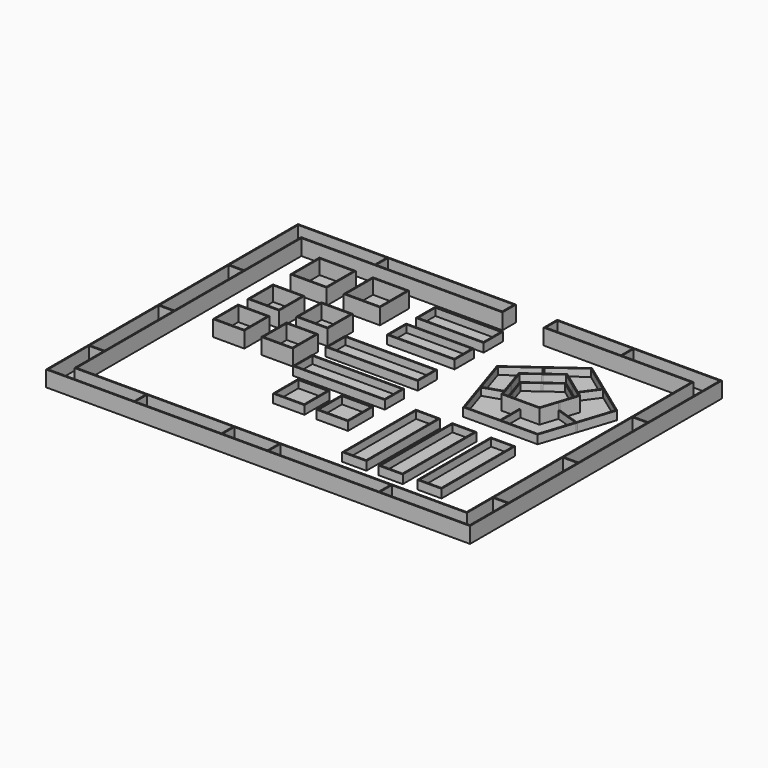
from build123d import *

# Parameters (mm, degrees)
F1_W     = 14
F1_H     = 14
F3_DEPTH = 6
F1_W_2   = 12
F1_H_2   = 12
F0_W     = 6
F0_H     = 0.5
F0_W_2   = 0.5
F0_H_2   = 6
F0_H_3   = 35.5
F0_W_3   = 52
F0_W_4   = 35.5
F0_W_5   = 18.5
F0_W_6   = 45.5
F0_W_7   = 31
F4_T     = 0.5
F4_2_T   = 0.5
F4_3_T   = 0.5
F4_4_T   = 0.5
F4_5_T   = 0.5
F4_6_T   = 0.5
F4_7_T   = 0.5
F4_8_T   = 0.5
F1_W_3   = 27
F1_H_3   = 9
F5_DEPTH = 3
F1_W_4   = 37
F1_W_5   = 9
F1_H_4   = 37
F2_W     = 0.5
F2_H     = 10.322864
F6_T     = 0.5
F6_2_T   = 0.5
F6_3_T   = 0.5
F6_4_T   = 0.5
F6_5_T   = 0.5
F6_6_T   = 0.5
F6_7_T   = 0.5
F6_8_T   = 0.5
F6_9_T   = 0.5
F6_10_T  = 0.5
F7_DEPTH = 6
F8_DEPTH = 3


with BuildPart() as f3:
    # F1 (on Top) → F3 (new body)
    with BuildSketch(Plane.XY):
        with Locations((-36.439199, 38.914477)):
            Rectangle(F1_W, F1_H)
    extrude(amount=F3_DEPTH)

    # F4#3
    f4_3_openings = [f3.faces().sort_by_distance(p)[0] for p in [
        (-36.439199, 38.914477, 6),
    ]]
    offset(amount=F4_3_T, openings=f4_3_openings, kind=Kind.INTERSECTION)


with BuildPart() as f3b:
    # F1 (on Top) → F3, piece 2 (new body)
    with BuildSketch(Plane.XY):
        with Locations((-58.439199, 38.914477)):
            Rectangle(F1_W, F1_H)
    extrude(amount=F3_DEPTH)

    # F4#2
    f4_2_openings = [f3b.faces().sort_by_distance(p)[0] for p in [
        (-58.439199, 38.914477, 6),
    ]]
    offset(amount=F4_2_T, openings=f4_2_openings, kind=Kind.INTERSECTION)


with BuildPart() as f3c:
    # F1 (on Top) → F3, piece 3 (new body)
    with BuildSketch(Plane.XY):
        with Locations((-59.439199, 15.914477)):
            Rectangle(F1_W_2, F1_H_2)
    extrude(amount=F3_DEPTH)

    # F4#5
    f4_5_openings = [f3c.faces().sort_by_distance(p)[0] for p in [
        (-59.439199, 15.914477, 6),
    ]]
    offset(amount=F4_5_T, openings=f4_5_openings, kind=Kind.INTERSECTION)


with BuildPart() as f3d:
    # F1 (on Top) → F3, piece 4 (new body)
    with BuildSketch(Plane.XY):
        with Locations((-59.439199, -2.085523)):
            Rectangle(F1_W_2, F1_H_2)
    extrude(amount=F3_DEPTH)

    # F4#6
    f4_6_openings = [f3d.faces().sort_by_distance(p)[0] for p in [
        (-59.439199, -2.085523, 6),
    ]]
    offset(amount=F4_6_T, openings=f4_6_openings, kind=Kind.INTERSECTION)


with BuildPart() as f3e:
    # F1 (on Top) → F3, piece 5 (new body)
    with BuildSketch(Plane.XY):
        with Locations((-39.439199, -2.085523)):
            Rectangle(F1_W_2, F1_H_2)
    extrude(amount=F3_DEPTH)

    # F4#7
    f4_7_openings = [f3e.faces().sort_by_distance(p)[0] for p in [
        (-39.439199, -2.085523, 6),
    ]]
    offset(amount=F4_7_T, openings=f4_7_openings, kind=Kind.INTERSECTION)


with BuildPart() as f3f:
    # F1 (on Top) → F3, piece 6 (new body)
    with BuildSketch(Plane.XY):
        with Locations((-39.439199, 15.914477)):
            Rectangle(F1_W_2, F1_H_2)
    extrude(amount=F3_DEPTH)

    # F4#4
    f4_4_openings = [f3f.faces().sort_by_distance(p)[0] for p in [
        (-39.439199, 15.914477, 6),
    ]]
    offset(amount=F4_4_T, openings=f4_4_openings, kind=Kind.INTERSECTION)


with BuildPart() as f3g:
    # F0 (on Top) → F3, piece 7 (new body)
    with BuildSketch(Plane.XY):
        Polygon((-48.945705, 59.870679), (-85.445705, 59.870679), (-85.445705, 24.370679), (-79.445705, 24.370679), (-79.445705, 53.870679), (-48.945705, 53.870679), align=None)
        with Locations((-82.445705, 24.120679)):
            Rectangle(F0_W, F0_H)
        with Locations((-48.695705, 56.870679)):
            Rectangle(F0_W_2, F0_H_2)
        with Locations((-82.445705, 6.120679)):
            Rectangle(F0_W, F0_H_3)
        with Locations((-22.445705, 56.870679)):
            Rectangle(F0_W_3, F0_H_2)
        with Locations((-82.445705, -11.879321)):
            Rectangle(F0_W, F0_H)
        with Locations((-82.445705, -29.879321)):
            Rectangle(F0_W, F0_H_3)
        with Locations((-82.445705, -47.879321)):
            Rectangle(F0_W, F0_H)
        Polygon((-79.445705, -48.129321), (-85.445705, -48.129321), (-85.445705, -69.129321), (-49.945705, -69.129321), (-49.945705, -63.129321), (-79.13054, -63.129321), (-79.445705, -63.129321), align=None)
        with Locations((-49.695705, -66.129321)):
            Rectangle(F0_W_2, F0_H_2)
        with Locations((-31.695705, -66.129321)):
            Rectangle(F0_W_4, F0_H_2)
        with Locations((-13.695705, -66.129321)):
            Rectangle(F0_W_2, F0_H_2)
        with Locations((-4.195705, -66.129321)):
            Rectangle(F0_W_5, F0_H_2)
        with Locations((5.304295, -66.129321)):
            Rectangle(F0_W_2, F0_H_2)
        with Locations((28.304295, -66.129321)):
            Rectangle(F0_W_6, F0_H_2)
        with Locations((51.304295, -66.129321)):
            Rectangle(F0_W_2, F0_H_2)
        Polygon((51.554295, -63.129321), (51.554295, -69.129321), (88.554295, -69.129321), (88.554295, -49.629321), (82.554295, -49.629321), (82.554295, -63.129321), align=None)
        with Locations((85.554295, -49.379321)):
            Rectangle(F0_W, F0_H)
        with Locations((85.554295, -31.379321)):
            Rectangle(F0_W, F0_H_3)
        with Locations((85.554295, -13.379321)):
            Rectangle(F0_W, F0_H)
        with Locations((85.554295, 4.620679)):
            Rectangle(F0_W, F0_H_3)
        with Locations((85.554295, 22.620679)):
            Rectangle(F0_W, F0_H)
        Polygon((82.554295, 22.870679), (88.554295, 22.870679), (88.554295, 59.870679), (53.054295, 59.870679), (53.054295, 53.870679), (82.554295, 53.870679), align=None)
        with Locations((52.804295, 56.870679)):
            Rectangle(F0_W_2, F0_H_2)
        with Locations((37.054295, 56.870679)):
            Rectangle(F0_W_7, F0_H_2)
    extrude(amount=F3_DEPTH)

    # F4
    f4_openings = [f3g.faces().sort_by_distance(p)[0] for p in [
        (-83.279671, -4.629321, 6),
    ]]
    offset(amount=F4_T, openings=f4_openings, kind=Kind.INTERSECTION)

    # F0 (on Top) → F7 (join)
    with BuildSketch(Plane.XY):
        with Locations((-48.695705, 56.870679)):
            Rectangle(F0_W_2, F0_H_2)
        with Locations((-82.445705, 24.120679)):
            Rectangle(F0_W, F0_H)
        with Locations((-82.445705, -11.879321)):
            Rectangle(F0_W, F0_H)
        with Locations((-82.445705, -47.879321)):
            Rectangle(F0_W, F0_H)
        with Locations((-49.695705, -66.129321)):
            Rectangle(F0_W_2, F0_H_2)
        with Locations((-13.695705, -66.129321)):
            Rectangle(F0_W_2, F0_H_2)
        with Locations((5.304295, -66.129321)):
            Rectangle(F0_W_2, F0_H_2)
        with Locations((51.304295, -66.129321)):
            Rectangle(F0_W_2, F0_H_2)
        with Locations((85.554295, -49.379321)):
            Rectangle(F0_W, F0_H)
        with Locations((85.554295, -13.379321)):
            Rectangle(F0_W, F0_H)
        with Locations((85.554295, 22.620679)):
            Rectangle(F0_W, F0_H)
        with Locations((52.804295, 56.870679)):
            Rectangle(F0_W_2, F0_H_2)
    extrude(amount=F7_DEPTH)


with BuildPart() as f3h:
    # F2 (on Top) → F3, piece 8 (new body)
    with BuildSketch(Plane.XY):
        Polygon((46.768948, 9.115655), (47.268948, 9.115655), (54.768948, 9.115655), (56.932067, 15.773051), (57.086575, 16.248579), (59.404203, 23.381503), (53.336575, 27.789892), (52.932067, 28.083785), (47.268948, 32.198282), (41.20132, 27.789892), (40.796812, 27.496), (35.133693, 23.381503), (37.45132, 16.248579), (37.605829, 15.773051), (39.768948, 9.115655), align=None)
    extrude(amount=F3_DEPTH)

    # F4#8
    f4_8_openings = [f3h.faces().sort_by_distance(p)[0] for p in [
        (47.268948, 19.43852, 6),
    ]]
    offset(amount=F4_8_T, openings=f4_8_openings, kind=Kind.INTERSECTION)


with BuildPart() as f5:
    # F1 (on Top) → F5 (new body)
    with BuildSketch(Plane.XY):
        with Locations((-4.939199, 42.414477)):
            Rectangle(F1_W_3, F1_H_3)
    extrude(amount=F5_DEPTH)

    # F6
    f6_openings = [f5.faces().sort_by_distance(p)[0] for p in [
        (-4.939199, 42.414477, 3),
    ]]
    offset(amount=F6_T, openings=f6_openings, kind=Kind.INTERSECTION)


with BuildPart() as f5b:
    # F1 (on Top) → F5, piece 2 (new body)
    with BuildSketch(Plane.XY):
        with Locations((-4.939199, 27.414477)):
            Rectangle(F1_W_3, F1_H_3)
    extrude(amount=F5_DEPTH)

    # F6#2
    f6_2_openings = [f5b.faces().sort_by_distance(p)[0] for p in [
        (-4.939199, 27.414477, 3),
    ]]
    offset(amount=F6_2_T, openings=f6_2_openings, kind=Kind.INTERSECTION)


with BuildPart() as f5c:
    # F1 (on Top) → F5, piece 3 (new body)
    with BuildSketch(Plane.XY):
        with Locations((-9.939199, 8.414477)):
            Rectangle(F1_W_4, F1_H_3)
    extrude(amount=F5_DEPTH)

    # F6#3
    f6_3_openings = [f5c.faces().sort_by_distance(p)[0] for p in [
        (-9.939199, 8.414477, 3),
    ]]
    offset(amount=F6_3_T, openings=f6_3_openings, kind=Kind.INTERSECTION)


with BuildPart() as f5d:
    # F1 (on Top) → F5, piece 4 (new body)
    with BuildSketch(Plane.XY):
        with Locations((-9.939199, -8.585523)):
            Rectangle(F1_W_4, F1_H_3)
    extrude(amount=F5_DEPTH)

    # F6#4
    f6_4_openings = [f5d.faces().sort_by_distance(p)[0] for p in [
        (-9.939199, -8.585523, 3),
    ]]
    offset(amount=F6_4_T, openings=f6_4_openings, kind=Kind.INTERSECTION)


with BuildPart() as f5e:
    # F1 (on Top) → F5, piece 5 (new body)
    with BuildSketch(Plane.XY):
        with Locations((-15.439199, -26.085523)):
            Rectangle(F1_W_2, F1_H_2)
    extrude(amount=F5_DEPTH)

    # F6#5
    f6_5_openings = [f5e.faces().sort_by_distance(p)[0] for p in [
        (-15.439199, -26.085523, 3),
    ]]
    offset(amount=F6_5_T, openings=f6_5_openings, kind=Kind.INTERSECTION)


with BuildPart() as f5f:
    # F1 (on Top) → F5, piece 6 (new body)
    with BuildSketch(Plane.XY):
        with Locations((2.560801, -26.085523)):
            Rectangle(F1_W_2, F1_H_2)
    extrude(amount=F5_DEPTH)

    # F6#6
    f6_6_openings = [f5f.faces().sort_by_distance(p)[0] for p in [
        (2.560801, -26.085523, 3),
    ]]
    offset(amount=F6_6_T, openings=f6_6_openings, kind=Kind.INTERSECTION)


with BuildPart() as f5g:
    # F1 (on Top) → F5, piece 7 (new body)
    with BuildSketch(Plane.XY):
        with Locations((26.060801, -31.585523)):
            Rectangle(F1_W_5, F1_H_4)
    extrude(amount=F5_DEPTH)

    # F6#7
    f6_7_openings = [f5g.faces().sort_by_distance(p)[0] for p in [
        (26.060801, -31.585523, 3),
    ]]
    offset(amount=F6_7_T, openings=f6_7_openings, kind=Kind.INTERSECTION)


with BuildPart() as f5h:
    # F1 (on Top) → F5, piece 8 (new body)
    with BuildSketch(Plane.XY):
        with Locations((41.060801, -31.585523)):
            Rectangle(F1_W_5, F1_H_4)
    extrude(amount=F5_DEPTH)

    # F6#8
    f6_8_openings = [f5h.faces().sort_by_distance(p)[0] for p in [
        (41.060801, -31.585523, 3),
    ]]
    offset(amount=F6_8_T, openings=f6_8_openings, kind=Kind.INTERSECTION)


with BuildPart() as f5i:
    # F1 (on Top) → F5, piece 9 (new body)
    with BuildSketch(Plane.XY):
        with Locations((57.060801, -31.585523)):
            Rectangle(F1_W_5, F1_H_4)
    extrude(amount=F5_DEPTH)

    # F6#9
    f6_9_openings = [f5i.faces().sort_by_distance(p)[0] for p in [
        (57.060801, -31.585523, 3),
    ]]
    offset(amount=F6_9_T, openings=f6_9_openings, kind=Kind.INTERSECTION)


with BuildPart() as f5j:
    # F2 (on Top) → F5, piece 10 (new body)
    with BuildSketch(Plane.XY):
        Polygon((22.998438, 27.324486), (27.633693, 13.058639), (37.45132, 16.248579), (35.133693, 23.381503), (40.796812, 27.496), (34.729184, 35.847373), align=None)
        Polygon((52.932067, 28.083785), (58.999694, 36.435158), (47.268948, 44.958044), (35.133693, 36.141265), (41.20132, 27.789892), (47.268948, 32.198282), align=None)
        Polygon((57.086575, 16.248579), (66.904203, 13.058639), (71.539458, 27.324486), (59.404203, 36.141265), (53.336575, 27.789892), (59.404203, 23.381503), align=None)
        Polygon((56.932067, 15.773051), (66.749694, 12.58311), (66.904203, 13.058639), (57.086575, 16.248579), align=None)
        Polygon((27.633693, 13.058639), (27.788201, 12.58311), (37.605829, 15.773051), (37.45132, 16.248579), align=None)
        Polygon((32.268948, -1.207209), (46.768948, -1.207209), (46.768948, 9.115655), (39.768948, 9.115655), (37.605829, 15.773051), (27.788201, 12.58311), align=None)
        Polygon((47.268948, -1.207209), (62.268948, -1.207209), (66.749694, 12.58311), (56.932067, 15.773051), (54.768948, 9.115655), (47.268948, 9.115655), align=None)
        with Locations((47.018948, 3.954223)):
            Rectangle(F2_W, F2_H)
        Polygon((53.336575, 27.789892), (59.404203, 36.141265), (58.999694, 36.435158), (52.932067, 28.083785), align=None)
        Polygon((35.133693, 36.141265), (34.729184, 35.847373), (40.796812, 27.496), (41.20132, 27.789892), align=None)
    extrude(amount=F5_DEPTH)

    # F6#10
    f6_10_openings = [f5j.faces().sort_by_distance(p)[0] for p in [
        (28.270792, 13.265645, 3),
    ]]
    offset(amount=F6_10_T, openings=f6_10_openings, kind=Kind.INTERSECTION)


with BuildPart() as f8:
    # F2 (on Top) → F8 (new body)
    with BuildSketch(Plane.XY):
        Polygon((27.633693, 13.058639), (27.788201, 12.58311), (37.605829, 15.773051), (37.45132, 16.248579), align=None)
    extrude(amount=F8_DEPTH)


with BuildPart() as f8b:
    # F2 (on Top) → F8, piece 2 (new body)
    with BuildSketch(Plane.XY):
        with Locations((47.018948, 3.954223)):
            Rectangle(F2_W, F2_H)
    extrude(amount=F8_DEPTH)


with BuildPart() as f8c:
    # F2 (on Top) → F8, piece 3 (new body)
    with BuildSketch(Plane.XY):
        Polygon((56.932067, 15.773051), (66.749694, 12.58311), (66.904203, 13.058639), (57.086575, 16.248579), align=None)
    extrude(amount=F8_DEPTH)


with BuildPart() as f8d:
    # F2 (on Top) → F8, piece 4 (new body)
    with BuildSketch(Plane.XY):
        Polygon((53.336575, 27.789892), (59.404203, 36.141265), (58.999694, 36.435158), (52.932067, 28.083785), align=None)
    extrude(amount=F8_DEPTH)


with BuildPart() as f8e:
    # F2 (on Top) → F8, piece 5 (new body)
    with BuildSketch(Plane.XY):
        Polygon((35.133693, 36.141265), (34.729184, 35.847373), (40.796812, 27.496), (41.20132, 27.789892), align=None)
    extrude(amount=F8_DEPTH)


solid = Compound([f3.part, f3b.part, f3c.part, f3d.part, f3e.part, f3f.part, f3g.part, f3h.part, f5.part, f5b.part, f5c.part, f5d.part, f5e.part, f5f.part, f5g.part, f5h.part, f5i.part, f5j.part, f8.part, f8b.part, f8c.part, f8d.part, f8e.part])
